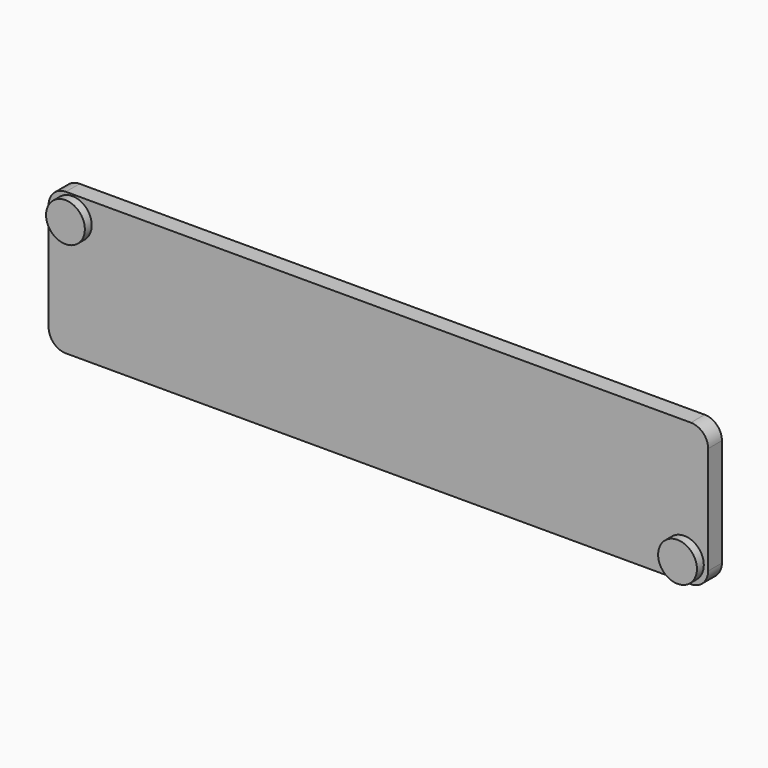
from build123d import *

# Parameters (mm, degrees)
F0_W     = 76.5
F0_H     = 16.5
F2_DEPTH = 2
F1_R     = 2.25
F3_DEPTH = 1
F4_R     = 2


with BuildPart() as f2:
    # F0 (on Front) → F2 (new body)
    with BuildSketch(Plane.XZ):
        Rectangle(F0_W, F0_H)
    extrude(amount=-F2_DEPTH)

    # F1 (on Front) → F3 (join)
    with BuildSketch(Plane.XZ):
        with Locations((-35.5, 5.8)):
            Circle(F1_R)
        with Locations((35.5, -5.8)):
            Circle(F1_R)
    extrude(amount=F3_DEPTH)

    # F4
    f4_edges = [f2.edges().sort_by_distance(p)[0] for p in [
        (38.25, 1, -8.25),
        (38.25, 1, 8.25),
        (-38.25, 1, -8.25),
        (-38.25, 1, 8.25),
    ]]
    fillet(f4_edges, radius=F4_R)


solid = f2.part
